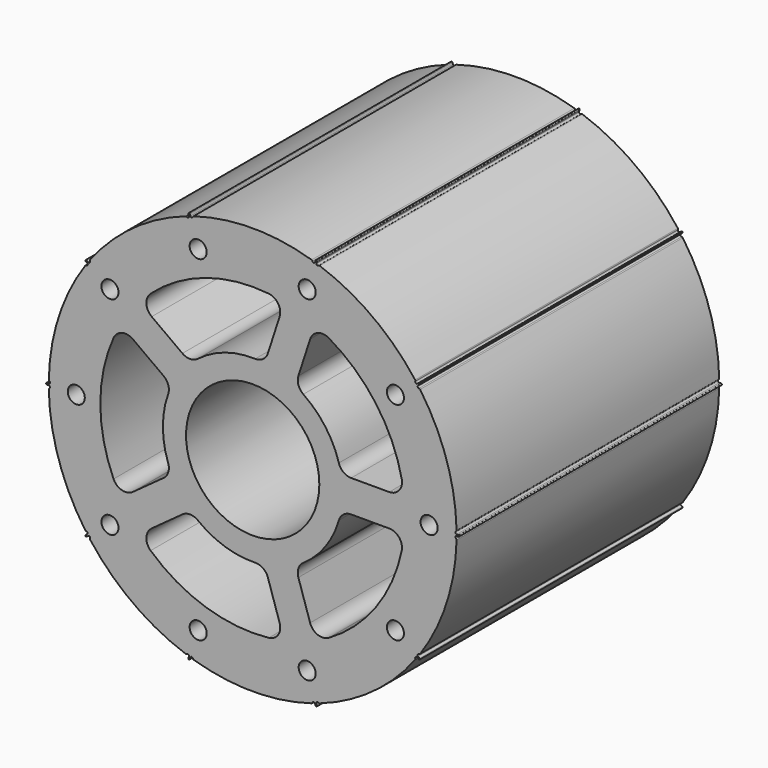
from build123d import *

# Parameters (mm, degrees)
F1_DEPTH        = 130
F2_R            = 26.391
F3_DEPTH        = 130
F4_D            = 6.7564
F6_DEPTH        = 130
F6_COPIES_COUNT = 5
F7_R            = 5.08


# Not quite as in the source:
# - a pattern or mirror of a feature is missing from the dataset's text; its kind, count and spacing are read off the source's solid


with BuildPart() as f1:
    # F0 (on Front) → F1 (new body)
    with BuildSketch(Plane.XZ):
        with BuildLine():
            ThreePointArc((23.7036118773, 76.9298434376), (23.5816837061, 77.1596187003), (23.3608317089, 77.2970506673))
            ThreePointArc((23.3608317089, 77.2970506673), (-0.0001147149, 80.75), (-23.361051328, 77.2969842934))
            ThreePointArc((-23.361051328, 77.2969842934), (-23.5811818782, 77.1603225108), (-23.7033557347, 76.9318330127))
            ThreePointArc((-23.7033557347, 76.9318330127), (-24.1707219857, 76.5456761593), (-24.6669025773, 76.8940339476))
            Line((-24.6669025773, 76.8940339476), (-24.8986653231, 77.6073263348))
            ThreePointArc((-24.8986653231, 77.6073263348), (-25.2766873763, 77.7999381914), (-25.4692992328, 77.4219161382))
            Line((-25.4692992328, 77.4219161382), (-25.237536487, 76.7086237509))
            ThreePointArc((-25.237536487, 76.7086237509), (-25.4350730727, 76.1345635963), (-26.0408720416, 76.174229364))
            ThreePointArc((-26.0408720416, 76.174229364), (-26.2745725149, 76.2884538755), (-26.5340260173, 76.2698251255))
            ThreePointArc((-26.5340260173, 76.2698251255), (-47.4630213735, 65.3321000288), (-64.3327843897, 48.8073376194))
            ThreePointArc((-64.3327843897, 48.8073376194), (-64.4305459654, 48.5673864238), (-64.3950839344, 48.3107225458))
            ThreePointArc((-64.3950839344, 48.3107225458), (-64.5462138705, 47.7236040991), (-65.1523919718, 47.7137838357))
            Line((-65.1523919718, 47.7137838357), (-65.7591547176, 48.154622775))
            ThreePointArc((-65.7591547176, 48.154622775), (-66.1781953916, 48.0882532523), (-66.111825869, 47.6692125783))
            Line((-66.111825869, 47.6692125783), (-65.5050631232, 47.2283736391))
            ThreePointArc((-65.5050631232, 47.2283736391), (-65.3274494852, 46.6478401264), (-65.8408660995, 46.3238507067))
            ThreePointArc((-65.8408660995, 46.3238507067), (-66.0970732373, 46.2788945861), (-66.2960258255, 46.1113206684))
            ThreePointArc((-66.2960258255, 46.1113206684), (-76.7989052383, 24.9607603697), (-80.7338185677, 1.6761488419))
            ThreePointArc((-80.7338185677, 1.6761488419), (-80.6718695698, 1.4245614344), (-80.4923169417, 1.2377600541))
            ThreePointArc((-80.4923169417, 1.2377600541), (-80.2694840641, 0.6739393053), (-80.7541202437, 0.3096919972))
            Line((-80.7541202437, 0.3096919972), (-81.5041202437, 0.3096919972))
            ThreePointArc((-81.5041202437, 0.3096919972), (-81.8041202437, 0.0096919972), (-81.5041202437, -0.2903080028))
            Line((-81.5041202437, -0.2903080028), (-80.7541202437, -0.2903080028))
            ThreePointArc((-80.7541202437, -0.2903080028), (-80.2691987549, -0.6555708034), (-80.4941253183, -1.219462464))
            ThreePointArc((-80.4941253183, -1.219462464), (-80.6749767021, -1.4064275067), (-80.7374352495, -1.6589390512))
            ThreePointArc((-80.7374352495, -1.6589390512), (-76.8024557631, -24.9435393989), (-66.2995162565, -46.0940698564))
            ThreePointArc((-66.2995162565, -46.0940698564), (-66.1015190967, -46.2611956373), (-65.8464588727, -46.3067827417))
            ThreePointArc((-65.8464588727, -46.3067827417), (-65.3347777668, -46.63194543), (-65.5127574763, -47.2114896916))
            Line((-65.5127574763, -47.2114896916), (-66.119520222, -47.6523286308))
            ThreePointArc((-66.119520222, -47.6523286308), (-66.1858897447, -48.0713693048), (-65.7668490707, -48.1377388274))
            Line((-65.7668490707, -48.1377388274), (-65.1600863249, -47.6968998882))
            ThreePointArc((-65.1600863249, -47.6968998882), (-64.5530805121, -47.7073740016), (-64.4036027223, -48.2957804549))
            ThreePointArc((-64.4036027223, -48.2957804549), (-64.4400192705, -48.5533401281), (-64.342126735, -48.7943384719))
            ThreePointArc((-64.342126735, -48.7943384719), (-47.472316768, -65.3190529502), (-26.5432903353, -76.2567185827))
            ThreePointArc((-26.5432903353, -76.2567185827), (-26.2848731988, -76.275546369), (-26.0517297154, -76.1625064731))
            ThreePointArc((-26.0517297154, -76.1625064731), (-25.4466451721, -76.124810006), (-25.2499862118, -76.698285011))
            Line((-25.2499862118, -76.698285011), (-25.4817489576, -77.4115773982))
            ThreePointArc((-25.4817489576, -77.4115773982), (-25.289137101, -77.7895994514), (-24.9111150478, -77.5969875949))
            Line((-24.9111150478, -77.5969875949), (-24.679352302, -76.8836952076))
            ThreePointArc((-24.679352302, -76.8836952076), (-24.1821177544, -76.5353798786), (-23.7153310466, -76.9235498585))
            ThreePointArc((-23.7153310466, -76.9235498585), (-23.5934028755, -77.1533251211), (-23.3725508783, -77.2907570882))
            ThreePointArc((-23.3725508783, -77.2907570882), (-0.0116044544, -80.7437064208), (23.3493321587, -77.2906907142))
            ThreePointArc((23.3493321587, -77.2906907142), (23.5694627088, -77.1540289316), (23.6916365654, -76.9255394336))
            ThreePointArc((23.6916365654, -76.9255394336), (24.1590028164, -76.5393825802), (24.655183408, -76.8877403684))
            Line((24.655183408, -76.8877403684), (24.8869461537, -77.6010327556))
            ThreePointArc((24.8869461537, -77.6010327556), (25.2649682069, -77.7936446122), (25.4575800635, -77.415622559))
            Line((25.4575800635, -77.415622559), (25.2258173177, -76.7023301718))
            ThreePointArc((25.2258173177, -76.7023301718), (25.4233539034, -76.1282700171), (26.0291528723, -76.1679357848))
            ThreePointArc((26.0291528723, -76.1679357848), (26.2628533456, -76.2821602963), (26.522306848, -76.2635315464))
            ThreePointArc((26.522306848, -76.2635315464), (47.4513022041, -65.3258064496), (64.3210652204, -48.8010440403))
            ThreePointArc((64.3210652204, -48.8010440403), (64.4188267961, -48.5610928447), (64.383364765, -48.3044289667))
            ThreePointArc((64.383364765, -48.3044289667), (64.5344947012, -47.71731052), (65.1406728025, -47.7074902566))
            Line((65.1406728025, -47.7074902566), (65.7474355483, -48.1483291958))
            ThreePointArc((65.7474355483, -48.1483291958), (66.1664762223, -48.0819596732), (66.1001066997, -47.6629189992))
            Line((66.1001066997, -47.6629189992), (65.4933439539, -47.22208006))
            ThreePointArc((65.4933439539, -47.22208006), (65.3157303159, -46.6415465472), (65.8291469302, -46.3175571276))
            ThreePointArc((65.8291469302, -46.3175571276), (66.0853540679, -46.272601007), (66.2843066561, -46.1050270893))
            ThreePointArc((66.2843066561, -46.1050270893), (76.787186069, -24.9544667906), (80.7220993984, -1.6698552628))
            ThreePointArc((80.7220993984, -1.6698552628), (80.6601504005, -1.4182678553), (80.4805977724, -1.231466475))
            ThreePointArc((80.4805977724, -1.231466475), (80.2577648948, -0.6676457262), (80.7424010744, -0.3033984181))
            Line((80.7424010744, -0.3033984181), (81.4924010744, -0.3033984181))
            ThreePointArc((81.4924010744, -0.3033984181), (81.7924010744, -0.0033984181), (81.4924010744, 0.2966015819))
            Line((81.4924010744, 0.2966015819), (80.7424010744, 0.2966015819))
            ThreePointArc((80.7424010744, 0.2966015819), (80.2574795855, 0.6618643825), (80.4824061489, 1.2257560431))
            ThreePointArc((80.4824061489, 1.2257560431), (80.6632575328, 1.4127210859), (80.7257160802, 1.6652326303))
            ThreePointArc((80.7257160802, 1.6652326303), (76.7907365938, 24.949832978), (66.2877970872, 46.1003634355))
            ThreePointArc((66.2877970872, 46.1003634355), (66.0897999274, 46.2674892164), (65.8347397034, 46.3130763208))
            ThreePointArc((65.8347397034, 46.3130763208), (65.3230585975, 46.6382390092), (65.5010383069, 47.2177832707))
            Line((65.5010383069, 47.2177832707), (66.1078010527, 47.6586222099))
            ThreePointArc((66.1078010527, 47.6586222099), (66.2275213073, 47.9498138563), (66.0211672681, 48.1876026803))
            ThreePointArc((66.0211672681, 48.1876026803), (65.8829789289, 48.1973831385), (65.7551299013, 48.1440324066))
            Line((65.7551299013, 48.1440324066), (65.1483671556, 47.7031934673))
            ThreePointArc((65.1483671556, 47.7031934673), (64.5413613427, 47.7136675807), (64.391883553, 48.302074034))
            ThreePointArc((64.391883553, 48.302074034), (64.4283001012, 48.5596337072), (64.3304075656, 48.800632051))
            ThreePointArc((64.3304075656, 48.800632051), (47.4605975987, 65.3253465293), (26.5315711659, 76.2630121618))
            ThreePointArc((26.5315711659, 76.2630121618), (26.2731540295, 76.2818399482), (26.040010546, 76.1688000523))
            ThreePointArc((26.040010546, 76.1688000523), (25.4349260028, 76.1311035851), (25.2382670425, 76.7045785902))
            Line((25.2382670425, 76.7045785902), (25.4700297882, 77.4178709774))
            ThreePointArc((25.4700297882, 77.4178709774), (25.2774179317, 77.7958930306), (24.8993958785, 77.603281174))
            Line((24.8993958785, 77.603281174), (24.6676331327, 76.8899887868))
            ThreePointArc((24.6676331327, 76.8899887868), (24.170398585, 76.5416734577), (23.7036118773, 76.9298434376))
        make_face()
    extrude(amount=F1_DEPTH)

    # F2 (on face) → F3 (cut, through all)
    with BuildSketch(Plane.XZ.offset(130)):
        Circle(F2_R)
    extrude(amount=-F3_DEPTH, mode=Mode.SUBTRACT)

    # F4 (through all)
    with Locations(Plane.XZ.offset(130)):
        with Locations((21.5848370571, 66.4312976632), (-21.5848370571, 66.4312976632), (-56.5098370571, 41.0567998726), (-69.85, 0), (-56.5098370571, -41.0567998726), (-21.5848370571, -66.4312976632), (21.5848370571, -66.4312976632), (56.5098370571, -41.0567998726), (69.85, 0), (56.5098370571, 41.0567998726)):
            Hole(F4_D / 2)

    # F5 (on face) → F6 (cut, through all)
    with BuildSketch(Plane.XZ.offset(130)):
        with BuildLine():
            ThreePointArc((12.4986768937, 59.0160037694), (-18.6414501857, 57.3724843455), (-44.8003786791, 40.3984120382))
            Line((-44.8003786791, 40.3984120382), (-24.573808138, 25.7029483444))
            ThreePointArc((-24.573808138, 25.7029483444), (-10.98864432, 33.8195697195), (4.7728144229, 35.2382440324))
            Line((4.7728144229, 35.2382440324), (12.4986768937, 59.0160037694))
        make_face()
    f6 = extrude(amount=-F6_DEPTH, mode=Mode.SUBTRACT)

    # F6_copies: F6 ×5 about axis
    f6_copies_axis = Axis((0, 0, 0), (0, 1, 0))
    for i in range(1, F6_COPIES_COUNT):
        add(f6.rotate(f6_copies_axis, i * 360 / F6_COPIES_COUNT), mode=Mode.SUBTRACT)

    # F7
    f7_edges = [f1.edges().sort_by_distance(p)[0] for p in [
        (-44.800379, -65, 40.398412),
        (-24.573808, -65, 25.702948),
        (4.772814, -65, 35.238244),
        (12.498677, -65, 59.016004),
        (12.498677, -65, -59.016004),
        (4.772814, -65, -35.238244),
        (-44.800379, -65, -40.398412),
        (-24.573808, -65, -25.702948),
        (-52.265251, -65, -30.123896),
        (-32.038681, -65, -15.428433),
        (-32.038681, -65, 15.428433),
        (-52.265251, -65, 30.123896),
        (59.989859, -65, -6.35),
        (34.988442, -65, -6.35),
        (24.577095, -65, -55.091488),
        (16.851232, -65, -31.313728),
        (24.577095, -65, 55.091488),
        (16.851232, -65, 31.313728),
        (59.989859, -65, 6.35),
        (34.988442, -65, 6.35),
    ]]
    fillet(f7_edges, radius=F7_R)


solid = f1.part
